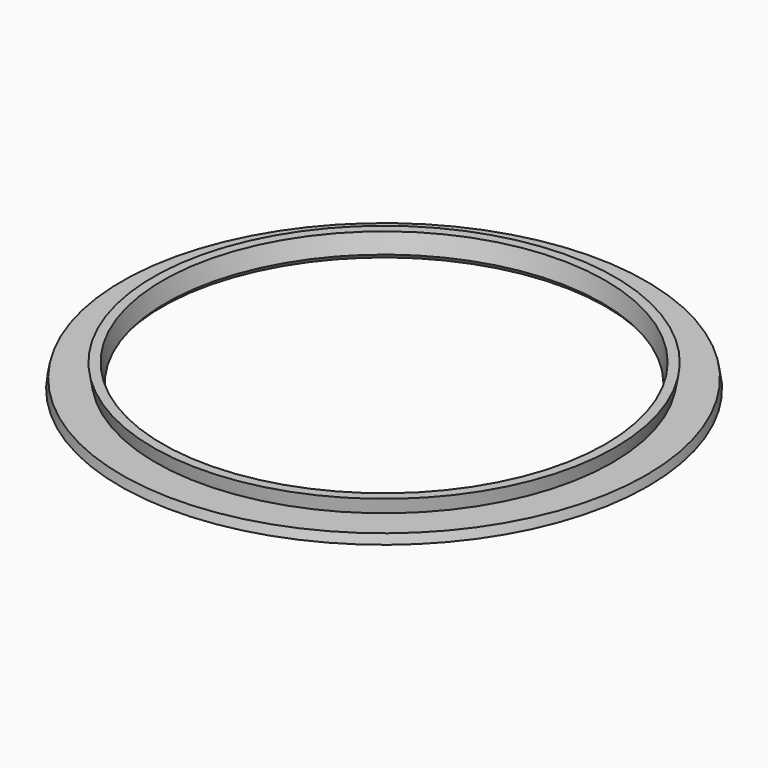
from build123d import *

# Parameters (mm, degrees)
F0_R     = 22.65
F0_R_2   = 18.65
F1_DEPTH = 2
F1_TAPER = 10
F2_T     = -0.8


# Not quite as in the source:
# - a fillet or chamfer that OpenCascade refuses, or shapes differently, is made with other operations: its cross-section is extruded or revolved along the edge and cut away or added


with BuildPart() as f1:
    # F0 (on Top) → F1 (new body)
    with BuildSketch(Plane.XY):
        Circle(F0_R)
        Circle(F0_R_2, mode=Mode.SUBTRACT)
    extrude(amount=F1_DEPTH, taper=F1_TAPER)

    # F2
    f2_openings = [f1.faces().sort_by_distance(p)[0] for p in [
        (-21.666682, 0, 2),
        (-22.473673, 0, 1),
    ]]
    offset(amount=F2_T, openings=f2_openings, kind=Kind.INTERSECTION)

    # F3: chamfer of 0.4 on 1 edges, made by hand

    # F3_s1 → F3_t2 (revolve, cut)
    with BuildSketch(Plane.XZ):
        Polygon((18.7194592711, 0.3939231012), (19.05, 0), (18.65, 0), align=None)
    revolve(axis=Axis((0, 0, 0), (0, 0, 1)), mode=Mode.SUBTRACT)


solid = f1.part
